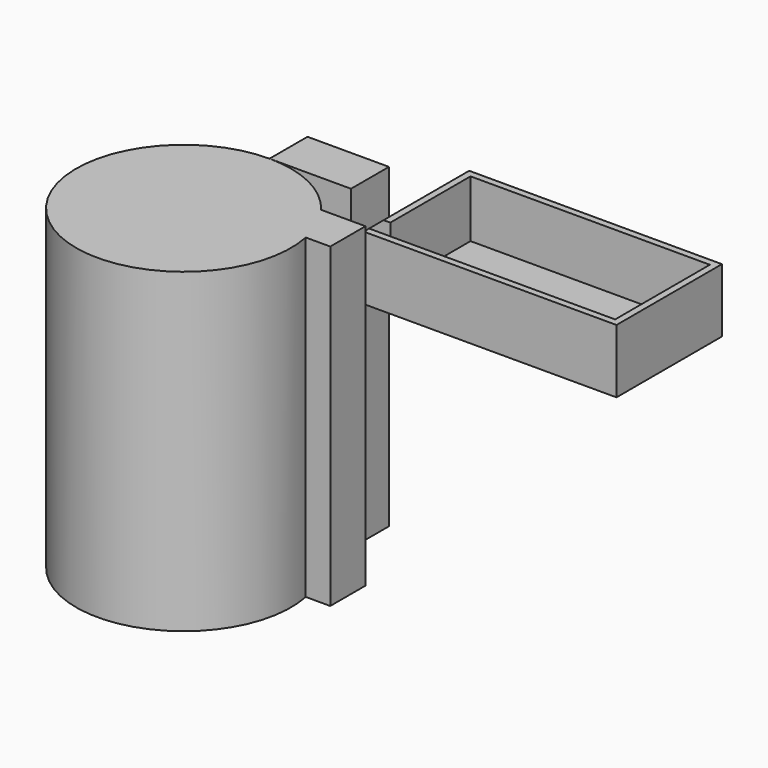
from build123d import *

# Parameters (mm, degrees)
F1_DEPTH = 119.888
F0_W     = 30.8635719121
F0_H     = 17.9806766311
F2_W     = 6.2429867685
F2_H     = 24.1485238075
F3_DEPTH = 95.758
F4_DEPTH = 43.688
F5_T     = -2.54


# Not quite as in the source:
# - a shell that OpenCascade refuses in one call is made with other operations: the cavity is built on its own and cut out


with BuildPart() as f1:
    # F0 (on Top) → F1 (new body)
    with BuildSketch(Plane.XY):
        with BuildLine():
            Line((49.202632159, 24.6388483793), (32.3984145703, 24.6388483793))
            ThreePointArc((32.3984145703, 24.6388483793), (18.0811546827, 36.4664498062), (0, 40.7029497227))
            ThreePointArc((0, 40.7029497227), (-25.8139115454, -31.4701777378), (39.9169293616, 7.9604564235))
            Line((39.9169293616, 7.9604564235), (49.202632159, 7.9604564235))
            Line((49.202632159, 7.9604564235), (49.202632159, 24.6388483793))
        make_face()
    extrude(amount=F1_DEPTH)


with BuildPart() as f1b:
    # F0 (on Top) → F1, piece 2 (new body)
    with BuildSketch(Plane.XY):
        with Locations((15.431785956, 49.6932880382)):
            Rectangle(F0_W, F0_H)
    extrude(amount=F1_DEPTH)

    # F2 (on face) → F3 (join)
    with BuildSketch(Plane.YZ.offset(30.8635719121)):
        with Locations((49.86118339, 91.0649970174)):
            Rectangle(F2_W, F2_H)
    extrude(amount=F3_DEPTH)

    # F4 (add): a face of the model
    f4_faces = [f1b.faces().sort_by_distance(p)[0] for p in [
        (78.7425719121, 52.9826767743, 91.0649970174),
    ]]
    extrude(f4_faces, amount=F4_DEPTH)

    # F5: a shell. OpenCascade refuses it in one call, so the cavity is built on its own and cut out:
    # the body offset inwards by the wall thickness, plus a prism from it out through each open face.
    f5_core = offset(f1b.part, amount=F5_T, kind=Kind.INTERSECTION, mode=Mode.PRIVATE)
    f5_exits = [f5_core.faces().sort_by_distance(p)[0] for p in [
        (78.335566, 71.543725, 100.599259),
    ]]
    add(f5_core, mode=Mode.SUBTRACT)
    extrude(f5_exits, amount=-F5_T, mode=Mode.SUBTRACT)


solid = Compound([f1.part, f1b.part])
